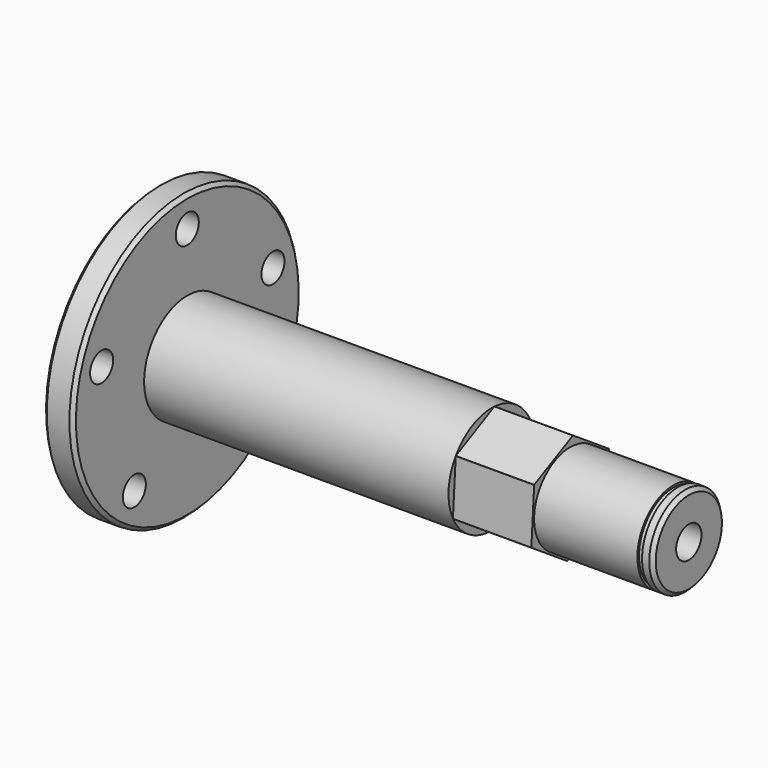
from build123d import *

# Parameters (mm, degrees)
F3_DEPTH  = 21.8
F4_R      = 12.5
F5_DEPTH  = 33
F6_SIZE   = 1
F6_2_SIZE = 1
F8_R      = 15
F8_R_2    = 11.95
F9_DEPTH  = 1.3
F10_R     = 4
F11_DEPTH = 8.3
F13_D     = 8.8
F13_DEPTH = 24
F13_TIP   = 2.6437867237


# Not quite as in the source:
# - two fillets or chamfers of one size are made in one step


with BuildPart() as f1:
    # F0 (on Front) → F1 (revolve)
    with BuildSketch(Plane.XZ):
        Polygon((0, 12.5), (0, 0), (107.9, 0), (107.9, 15), (23.3, 15), (23.3, 39.7), (15, 39.7), (15, 12.5), align=None)
    revolve(axis=Axis((53.95, 0, 0), (-1, 0, 0)))

    # F6#2
    f6_2_edges = [f1.edges().sort_by_distance(p)[0] for p in [
        (23.3, 0, -39.7),
        (15, 0, -39.7),
    ]]
    chamfer(f6_2_edges, length=F6_2_SIZE)

    # F10 (on face) → F11 (cut, through all)
    with BuildSketch(Plane.YZ.offset(23.3)):
        with Locations((0, 31.3)):
            Circle(F10_R)
        with Locations((29.76806896, 9.6722319239)):
            Circle(F10_R)
        with Locations((18.3976783968, -25.3222319239)):
            Circle(F10_R)
        with Locations((-18.3976783968, -25.3222319239)):
            Circle(F10_R)
        with Locations((-29.76806896, 9.6722319239)):
            Circle(F10_R)
    extrude(amount=-F11_DEPTH, mode=Mode.SUBTRACT)


with BuildPart() as f3:
    # F2 (on face) → F3 (new body)
    with BuildSketch(Plane.YZ.offset(107.9)):
        with BuildLine():
            Line((-0.9560760495, -14.9694996105), (12.4645414386, -8.3447712207))
            ThreePointArc((12.4645414386, -8.3447712207), (12.4752454622, -8.3287604515), (12.4859289198, -8.3127359521))
            Line((12.4859289198, -8.3127359521), (13.4590545852, 6.622223922))
            ThreePointArc((13.4590545852, 6.622223922), (13.4505408641, 6.6394992629), (13.4420049694, 6.6567636584))
            Line((13.4420049694, 6.6567636584), (0.9945131466, 14.9669951427))
            ThreePointArc((0.9945131466, 14.9669951427), (0.975295402, 14.9682597144), (0.9560760495, 14.9694996105))
            Line((0.9560760495, 14.9694996105), (-12.4645414386, 8.3447712207))
            ThreePointArc((-12.4645414386, 8.3447712207), (-12.4752454622, 8.3287604515), (-12.4859289198, 8.3127359521))
            Line((-12.4859289198, 8.3127359521), (-13.4590545852, -6.622223922))
            ThreePointArc((-13.4590545852, -6.622223922), (-13.4505408641, -6.6394992629), (-13.4420049694, -6.6567636584))
            Line((-13.4420049694, -6.6567636584), (-0.9945131466, -14.9669951427))
            ThreePointArc((-0.9945131466, -14.9669951427), (-0.975295402, -14.9682597144), (-0.9560760495, -14.9694996105))
        make_face()
    extrude(amount=F3_DEPTH)

    # F4 (on face) → F5 (join)
    with BuildSketch(Plane.YZ.offset(129.7)):
        Circle(F4_R)
    extrude(amount=F5_DEPTH)

    # F6
    f6_edges = [f3.edges().sort_by_distance(p)[0] for p in [
        (162.7, -12.5, 0),
    ]]
    chamfer(f6_edges, length=F6_SIZE)

    # F8 (on offset) → F9 (cut)
    with BuildSketch(Plane.YZ.offset(159.7)):
        Circle(F8_R)
        Circle(F8_R_2, mode=Mode.SUBTRACT)
    extrude(amount=-F9_DEPTH, mode=Mode.SUBTRACT)

    # F13
    with Locations(Plane.YZ.offset(162.7)):
        with Locations((0, 0)):
            Hole(F13_D / 2, depth=F13_DEPTH)
            with Locations((0, 0, -(F13_DEPTH + F13_TIP / 2))):  # 118° drill point
                Cone(0, F13_D / 2, F13_TIP, mode=Mode.SUBTRACT)


solid = Compound([f1.part, f3.part])
